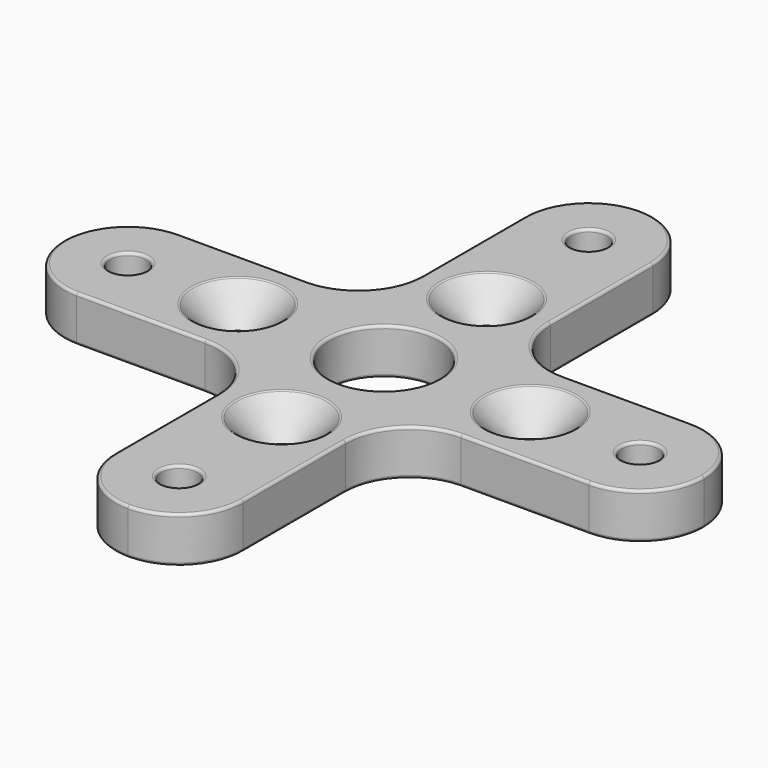
from build123d import *

# Parameters (mm, degrees)
F0_R     = 1
F0_R_2   = 0.8
F0_R_3   = 3
F1_DEPTH = 2.5
F2_R     = 3.49999
F3_SIZE  = 1.7
F4_R     = 0.15


# Not quite as in the source:
# - a fillet or chamfer is up to 0.001 mm smaller than in the source, because OpenCascade refuses the exact size


with BuildPart() as f1:
    # F0 (on Top) → F1 (new body)
    with BuildSketch(Plane.XY):
        Polygon((-24.8403990492, -37.8702705037), (-17.8403990492, -37.8702705037), (-17.8403990492, -23.8702705037), (-3.8403990492, -23.8702705037), (-3.8403990492, -16.8702705037), (-17.8403990492, -16.8702705037), (-17.8403990492, -2.8702705037), (-24.8403990492, -2.8702705037), (-24.8403990492, -16.8702705037), (-38.8403990492, -16.8702705037), (-38.8403990492, -23.8702705037), (-24.8403990492, -23.8702705037), align=None)
        with Locations((-21.3403990492, -34.3702705037)):
            Circle(F0_R, mode=Mode.SUBTRACT)
        with Locations((-21.3403990492, -27.3702705037)):
            Circle(F0_R_2, mode=Mode.SUBTRACT)
        with Locations((-35.3403990492, -20.3702705037)):
            Circle(F0_R, mode=Mode.SUBTRACT)
        with Locations((-29.3403990492, -20.3702705037)):
            Circle(F0_R_2, mode=Mode.SUBTRACT)
        with Locations((-21.3403990492, -13.3702705037)):
            Circle(F0_R_2, mode=Mode.SUBTRACT)
        with Locations((-21.3403990492, -6.3702705037)):
            Circle(F0_R, mode=Mode.SUBTRACT)
        with Locations((-21.3403990492, -20.3702705037)):
            Circle(F0_R_3, mode=Mode.SUBTRACT)
        with Locations((-13.3403990492, -20.3702705037)):
            Circle(F0_R_2, mode=Mode.SUBTRACT)
        with Locations((-7.3403990492, -20.3702705037)):
            Circle(F0_R, mode=Mode.SUBTRACT)
    extrude(amount=F1_DEPTH)

    # F2 (radius 3.5 in the source; OpenCascade refuses exactly that, so slightly less here)
    f2_edges = [f1.edges().sort_by_distance(p)[0] for p in [
        (-24.840399, -2.870271, 1.25),
        (-17.840399, -2.870271, 1.25),
        (-3.840399, -16.870271, 1.25),
        (-3.840399, -23.870271, 1.25),
        (-17.840399, -37.870271, 1.25),
        (-24.840399, -37.870271, 1.25),
        (-38.840399, -23.870271, 1.25),
        (-38.840399, -16.870271, 1.25),
        (-24.840399, -23.870271, 1.25),
        (-17.840399, -23.870271, 1.25),
        (-17.840399, -16.870271, 1.25),
        (-24.840399, -16.870271, 1.25),
    ]]
    fillet(f2_edges, radius=F2_R)

    # F3
    f3_edges = [f1.edges().sort_by_distance(p)[0] for p in [
        (-22.140399, -13.370271, 2.5),
        (-14.140399, -20.370271, 2.5),
        (-22.140399, -27.370271, 2.5),
        (-30.140399, -20.370271, 2.5),
    ]]
    chamfer(f3_edges, length=F3_SIZE)

    # F4
    f4_edges = [f1.edges().sort_by_distance(p)[0] for p in [
        (-23.840399, -13.370271, 2.5),
        (-31.840399, -23.870271, 2.5),
        (-37.815276, -22.845147, 2.5),
        (-25.865522, -24.895394, 2.5),
        (-38.840399, -20.370271, 2.5),
        (-24.840399, -30.870271, 2.5),
        (-37.815276, -17.895394, 2.5),
        (-23.815276, -36.845147, 2.5),
        (-31.840399, -16.870271, 2.5),
        (-21.340399, -37.870271, 2.5),
        (-25.865522, -15.845147, 2.5),
        (-18.865522, -36.845147, 2.5),
        (-24.840399, -9.870271, 2.5),
        (-17.840399, -30.870271, 2.5),
        (-23.815276, -3.895394, 2.5),
        (-16.815276, -24.895394, 2.5),
        (-21.340399, -2.870271, 2.5),
        (-10.840399, -23.870271, 2.5),
        (-18.865522, -3.895394, 2.5),
        (-4.865522, -22.845147, 2.5),
        (-17.840399, -9.870271, 2.5),
        (-3.840399, -20.370271, 2.5),
        (-16.815276, -15.845147, 2.5),
        (-4.865522, -17.895394, 2.5),
        (-10.840399, -16.870271, 2.5),
        (-22.340399, -34.370271, 2.5),
        (-36.340399, -20.370271, 2.5),
        (-22.340399, -6.370271, 2.5),
        (-24.340399, -20.370271, 2.5),
        (-8.340399, -20.370271, 2.5),
        (-15.840399, -20.370271, 2.5),
        (-23.840399, -27.370271, 2.5),
        (-31.840399, -20.370271, 2.5),
        (-31.840399, -23.870271, 0),
        (-37.815276, -22.845147, 0),
        (-25.865522, -24.895394, 0),
        (-38.840399, -20.370271, 0),
        (-24.840399, -30.870271, 0),
        (-37.815276, -17.895394, 0),
        (-23.815276, -36.845147, 0),
        (-31.840399, -16.870271, 0),
        (-21.340399, -37.870271, 0),
        (-25.865522, -15.845147, 0),
        (-18.865522, -36.845147, 0),
        (-24.840399, -9.870271, 0),
        (-17.840399, -30.870271, 0),
        (-23.815276, -3.895394, 0),
        (-16.815276, -24.895394, 0),
        (-21.340399, -2.870271, 0),
        (-10.840399, -23.870271, 0),
        (-18.865522, -3.895394, 0),
        (-4.865522, -22.845147, 0),
        (-17.840399, -9.870271, 0),
        (-3.840399, -20.370271, 0),
        (-16.815276, -15.845147, 0),
        (-4.865522, -17.895394, 0),
        (-10.840399, -16.870271, 0),
        (-22.340399, -34.370271, 0),
        (-22.140399, -27.370271, 0),
        (-36.340399, -20.370271, 0),
        (-30.140399, -20.370271, 0),
        (-22.140399, -13.370271, 0),
        (-22.340399, -6.370271, 0),
        (-24.340399, -20.370271, 0),
        (-14.140399, -20.370271, 0),
        (-8.340399, -20.370271, 0),
    ]]
    fillet(f4_edges, radius=F4_R)


solid = f1.part
